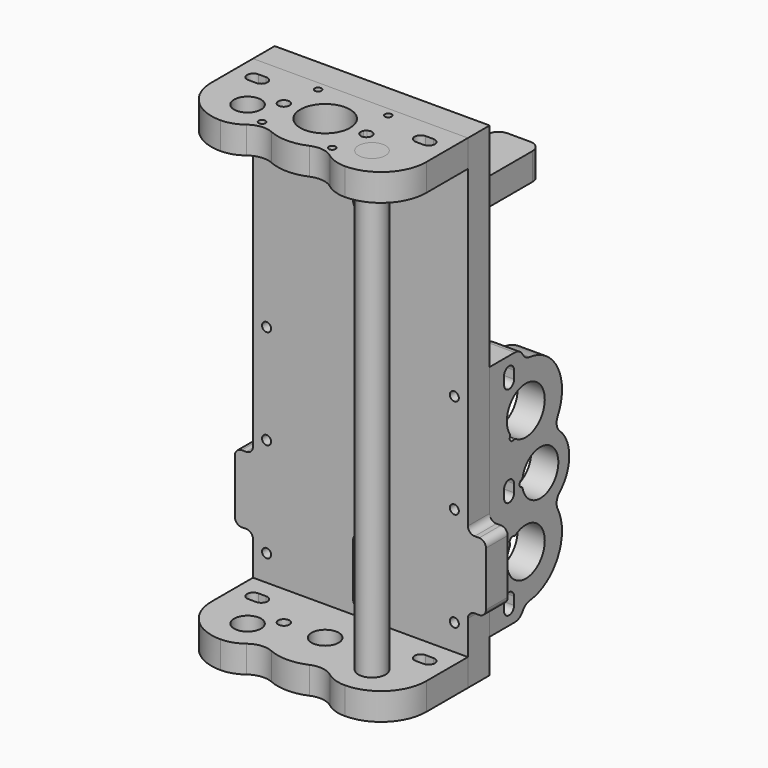
from build123d import *

# Parameters (mm, degrees)
F2_DEPTH       = 12
F3_R           = 11
F3_R_2         = 5.975
F4_DEPTH       = 12
F5_R           = 10
F6_R           = 6
F7_DEPTH       = 214
F9_DEPTH       = 12
F10_R          = 2.5
F10_R_2        = 6
F10_R_3        = 5.9749995874
F11_DEPTH      = 12
F12_R          = 2
F13_DEPTH      = 25
F13_DEPTH_BACK = 10
F14_R          = 1.5
F15_DEPTH      = 25
F16_R          = 5
F17_R          = 5
F18_W          = 8
F18_H          = 30
F19_DEPTH      = 12
F20_R          = 3
F21_W          = 20
F21_H          = 12
F22_DEPTH      = 59
F23_R          = 5


# Not quite as in the source:
# - ends of sketch curves that miss each other by under 0.0002 mm in the source are joined


with BuildPart() as f2:
    # F1 (on Front) → F2 (new body)
    with BuildSketch(Plane.XZ):
        Polygon((-47.5, 1.6334e-06), (47.5, -1.6334e-06), (47.5, 214.0000016334), (-47.5, 214.0000016334), align=None)
        with BuildLine():
            ThreePointArc((3.25, 18), (0, 14.75), (-3.25, 18))
            Line((-3.25, 18), (-3.25, 41))
            ThreePointArc((-3.25, 41), (0, 44.25), (3.25, 41))
            Line((3.25, 41), (3.25, 18))
        make_face(mode=Mode.SUBTRACT)
        with BuildLine():
            ThreePointArc((-3.25, 196.0000016334), (0, 199.2500016334), (3.25, 196.0000016334))
            Line((3.25, 196.0000016334), (3.25, 173.0000016334))
            ThreePointArc((3.25, 173.0000016334), (0, 169.7500016334), (-3.25, 173.0000016334))
            Line((-3.25, 173.0000016334), (-3.25, 196.0000016334))
        make_face(mode=Mode.SUBTRACT)
    extrude(amount=-F2_DEPTH)


with BuildPart() as f4:
    # F3 (on face) → F4 (new body)
    with BuildSketch(Plane.XY.offset(214.0000016334)):
        with BuildLine():
            Line((-7.7942286341, 0), (-47.5, 0))
            Line((-47.5, 0), (-47.5, -23))
            ThreePointArc((-47.5, -23), (-41.6421356237, -37.1421356237), (-27.5, -43))
            ThreePointArc((-27.5, -43), (-42.0543335736, -24.3707612055), (-20.4571797288, -14.7561832304))
            ThreePointArc((-20.4571797288, -14.7561832304), (-15.9364912858, -5.8241729502), (-7.7942286341, 0))
        make_face()
        with BuildLine():
            ThreePointArc((-38.75, -13.5), (-41.5, -10.75), (-38.75, -8))
            Line((-38.75, -8), (-35.25, -8))
            ThreePointArc((-35.25, -8), (-32.5, -10.75), (-35.25, -13.5))
            Line((-35.25, -13.5), (-38.75, -13.5))
        make_face(mode=Mode.SUBTRACT)
        with BuildLine():
            Line((7.7942286341, 0), (-7.7942286341, 0))
            ThreePointArc((-7.7942286341, 0), (-15.9364912858, -5.8241729502), (-20.4571797288, -14.7561832304))
            ThreePointArc((-20.4571797288, -14.7561832304), (-18.5664260205, -15.950466567), (-16.8742462967, -17.4125849124))
            ThreePointArc((-16.8742462967, -17.4125849124), (-16.4091811981, -17.8084367766), (-16.0539715251, -18.3052368697))
            ThreePointArc((-16.0539715251, -18.3052368697), (-13.4164914328, -22.8371726314), (-12.5, -28))
            ThreePointArc((-12.5, -28), (-12.9343908099, -31.5837171931), (-14.212403856, -34.9598698777))
            ThreePointArc((-14.212403856, -34.9598698777), (0, -40.5), (14.212403856, -34.9598698777))
            ThreePointArc((14.212403856, -34.9598698777), (12.5908669986, -26.3514390682), (16.0539715251, -18.3052368697))
            ThreePointArc((16.0539715251, -18.3052368697), (16.4091811981, -17.8084367766), (16.8742462967, -17.4125849124))
            ThreePointArc((16.8742462967, -17.4125849124), (18.5664260205, -15.950466567), (20.4571797288, -14.7561832304))
            ThreePointArc((20.4571797288, -14.7561832304), (15.9364912858, -5.8241729502), (7.7942286341, 0))
        make_face()
        with Locations((0, -19.5)):
            Circle(F3_R, mode=Mode.SUBTRACT)
        with BuildLine():
            Line((47.5, 0), (7.7942286341, 0))
            ThreePointArc((7.7942286341, 0), (15.9364912858, -5.8241729502), (20.4571797288, -14.7561832304))
            ThreePointArc((20.4571797288, -14.7561832304), (35.2252086034, -15.1422726723), (42.5, -28))
            ThreePointArc((42.5, -28), (38.1066017178, -38.6066017178), (27.5, -43))
            ThreePointArc((27.5, -43), (41.6421356237, -37.1421356237), (47.5, -23))
            Line((47.5, -23), (47.5, 0))
        make_face()
        with BuildLine():
            Line((38.75, -13.5), (35.25, -13.5))
            ThreePointArc((35.25, -13.5), (32.5, -10.75), (35.25, -8))
            Line((35.25, -8), (38.75, -8))
            ThreePointArc((38.75, -8), (41.5, -10.75), (38.75, -13.5))
        make_face(mode=Mode.SUBTRACT)
        with BuildLine():
            ThreePointArc((-16.8742462967, -17.4125849124), (-18.5664260205, -15.950466567), (-20.4571797288, -14.7561832304))
            ThreePointArc((-20.4571797288, -14.7561832304), (-20.0634554606, -25.7014316878), (-14.212403856, -34.9598698777))
            ThreePointArc((-14.212403856, -34.9598698777), (-12.9343908099, -31.5837171931), (-12.5, -28))
            ThreePointArc((-12.5, -28), (-13.4164914328, -22.8371726314), (-16.0539715251, -18.3052368697))
            ThreePointArc((-16.0539715251, -18.3052368697), (-15.8271843666, -18.8835874706), (-15.75, -19.5))
            ThreePointArc((-15.75, -19.5), (-20.4510661347, -20.6854568195), (-16.8742462967, -17.4125849124))
        make_face()
        with BuildLine():
            ThreePointArc((-14.212403856, -34.9598698777), (-20.0634554606, -25.7014316878), (-20.4571797288, -14.7561832304))
            ThreePointArc((-20.4571797288, -14.7561832304), (-42.0543335736, -24.3707612055), (-27.5, -43))
            ThreePointArc((-27.5, -43), (-19.7346296986, -40.8335117595), (-14.212403856, -34.9598698777))
        make_face()
        with Locations((-27.5, -28)):
            Circle(F3_R_2, mode=Mode.SUBTRACT)
        with BuildLine():
            ThreePointArc((42.5, -28), (35.2252086034, -15.1422726723), (20.4571797288, -14.7561832304))
            ThreePointArc((20.4571797288, -14.7561832304), (20.0634554606, -25.7014316878), (14.212403856, -34.9598698777))
            ThreePointArc((14.212403856, -34.9598698777), (19.7346296986, -40.8335117595), (27.5, -43))
            ThreePointArc((27.5, -43), (38.1066017178, -38.6066017178), (42.5, -28))
        make_face()
        with Locations((27.5, -28)):
            Circle(F3_R_2, mode=Mode.SUBTRACT)
        with BuildLine():
            ThreePointArc((14.212403856, -34.9598698777), (20.0634554606, -25.7014316878), (20.4571797288, -14.7561832304))
            ThreePointArc((20.4571797288, -14.7561832304), (18.5664260205, -15.950466567), (16.8742462967, -17.4125849124))
            ThreePointArc((16.8742462967, -17.4125849124), (19.4354568195, -17.2989338653), (20.75, -19.5))
            ThreePointArc((20.75, -19.5), (17.6335874706, -21.9228156334), (16.0539715251, -18.3052368697))
            ThreePointArc((16.0539715251, -18.3052368697), (12.5908669986, -26.3514390682), (14.212403856, -34.9598698777))
        make_face()
    extrude(amount=-F4_DEPTH)

    # F5
    f5_edges = [f4.edges().sort_by_distance(p)[0] for p in [
        (-14.212404, -34.95987, 208.000002),
        (14.212404, -34.95987, 208.000002),
    ]]
    fillet(f5_edges, radius=F5_R)


with BuildPart() as f7:
    # F6 (on face) → F7 (new body)
    with BuildSketch(Plane.XY.offset(214.0000016334)):
        with Locations((27.5, -28)):
            Circle(F6_R)
    extrude(amount=-F7_DEPTH)


with BuildPart() as f9:
    # F8 (on face) → F9 (new body)
    with BuildSketch(Plane.YZ.offset(47.5)):
        with BuildLine():
            Line((28.5, 14.9999964573), (32, 19.9999983666))
            ThreePointArc((32, 19.9999983666), (46.1421356237, 25.8578627429), (52, 39.9999983666))
            ThreePointArc((52, 39.9999983666), (50.7273420335, 47.0204442471), (47.071333964, 53.1474274897))
            ThreePointArc((47.071333964, 53.1474274897), (56, 67.4999964573), (47.071333964, 81.8525654249))
            ThreePointArc((47.071333964, 81.8525654249), (50.7273420335, 87.9795486675), (52, 94.9999945479))
            ThreePointArc((52, 94.9999945479), (46.1421356237, 109.1421301717), (32, 114.9999945479))
            Line((32, 114.9999945479), (28.5, 119.9999964573))
            Line((28.5, 119.9999964573), (12, 119.9999964573))
            Line((12, 119.9999964573), (12, 14.9999964573))
            Line((12, 14.9999964573), (28.5, 14.9999964573))
        make_face()
        with BuildLine():
            ThreePointArc((20, 25.2499964573), (22.75, 27.9999964573), (25.5, 25.2499964573))
            Line((25.5, 25.2499964573), (25.5, 21.7499964573))
            ThreePointArc((25.5, 21.7499964573), (22.75, 18.9999964573), (20, 21.7499964573))
            Line((20, 21.7499964573), (20, 25.2499964573))
        make_face(mode=Mode.SUBTRACT)
        with BuildLine():
            ThreePointArc((26.2943182564, 48.7846907824), (39.4069435329, 32.5930548337), (23.2153075842, 45.7056801102))
            ThreePointArc((23.2153075842, 45.7056801102), (23.3755438907, 46.2028582229), (23.2632266648, 46.7130019187))
            ThreePointArc((23.2632266648, 46.7130019187), (23.5323962953, 48.4676020713), (25.286996448, 48.7367717018))
            ThreePointArc((25.286996448, 48.7367717018), (25.7971401438, 48.6244544759), (26.2943182564, 48.7846907824))
        make_face(mode=Mode.SUBTRACT)
        with BuildLine():
            Line((20, 65.5727162957), (20, 69.0727162957))
            ThreePointArc((20, 69.0727162957), (22.75, 71.8227162957), (25.5, 69.0727162957))
            Line((25.5, 69.0727162957), (25.5, 65.5727162957))
            ThreePointArc((25.5, 65.5727162957), (22.75, 62.8227162957), (20, 65.5727162957))
        make_face(mode=Mode.SUBTRACT)
        with BuildLine():
            ThreePointArc((30.2641799544, 69.6712709771), (49.975, 67.4999964573), (30.2641799544, 65.3287219374))
            ThreePointArc((30.2641799544, 65.3287219374), (30.0228916348, 65.7894059146), (29.5828947368, 66.0666287667))
            ThreePointArc((29.5828947368, 66.0666287667), (28.525, 67.4999964573), (29.5828947368, 68.9333641478))
            ThreePointArc((29.5828947368, 68.9333641478), (30.0228916348, 69.210587), (30.2641799544, 69.6712709771))
        make_face(mode=Mode.SUBTRACT)
        with BuildLine():
            Line((25.5, 113.2499964573), (25.5, 109.7499964573))
            ThreePointArc((25.5, 109.7499964573), (22.75, 106.9999964573), (20, 109.7499964573))
            Line((20, 109.7499964573), (20, 113.2499964573))
            ThreePointArc((20, 113.2499964573), (22.75, 115.9999964573), (25.5, 113.2499964573))
        make_face(mode=Mode.SUBTRACT)
        with BuildLine():
            ThreePointArc((23.2632266648, 88.2869909959), (23.3755438907, 88.7971346917), (23.2153075842, 89.2943128043))
            ThreePointArc((23.2153075842, 89.2943128043), (39.4069435329, 102.4069380809), (26.2943182564, 86.2153021321))
            ThreePointArc((26.2943182564, 86.2153021321), (25.7971401438, 86.3755384387), (25.286996448, 86.2632212128))
            ThreePointArc((25.286996448, 86.2632212128), (23.5323962953, 86.5323908432), (23.2632266648, 88.2869909959))
        make_face(mode=Mode.SUBTRACT)
    extrude(amount=-F9_DEPTH)


with BuildPart() as f11:
    # F10 (on face) → F11 (new body)
    with BuildSketch(Plane(origin=(0, 0, 0), x_dir=(1, 0, -3.44e-08), z_dir=(-3.44e-08, 0, -1))):
        with BuildLine():
            Line((-47.5000069462, 23), (-47.5000069462, 0))
            Line((-47.5000069462, 0), (47.4999930538, 0))
            Line((47.4999930538, 0), (47.4999930538, 23))
            ThreePointArc((47.4999930538, 23), (41.6421286776, 37.1421356237), (27.4999930538, 43))
            ThreePointArc((27.4999930538, 43), (22.7171725023, 42.217054249), (18.4336441907, 39.9499508691))
            ThreePointArc((18.4336441907, 39.9499508691), (13.5760949869, 37.9872452657), (8.3928250358, 38.7499445297))
            ThreePointArc((8.3928250358, 38.7499445297), (-7.3588e-06, 40.5), (-8.3928397534, 38.7499445297))
            ThreePointArc((-8.3928397534, 38.7499445297), (-13.5761097045, 37.9872452657), (-18.4336589083, 39.9499508691))
            ThreePointArc((-18.4336589083, 39.9499508691), (-22.7171872199, 42.217054249), (-27.5000073588, 43))
            ThreePointArc((-27.5000073588, 43), (-41.6421425699, 37.1421356237), (-47.5000069462, 23))
        make_face()
        with BuildLine():
            Line((-35.2500069462, 8), (-38.7500069462, 8))
            ThreePointArc((-38.7500069462, 8), (-41.5000069462, 10.75), (-38.7500069462, 13.5))
            Line((-38.7500069462, 13.5), (-35.2500069462, 13.5))
            ThreePointArc((-35.2500069462, 13.5), (-32.5000069462, 10.75), (-35.2500069462, 8))
        make_face(mode=Mode.SUBTRACT)
        with Locations((-18.2500073588, 19.5)):
            Circle(F10_R, mode=Mode.SUBTRACT)
        with Locations((-7.3588e-06, 19.5)):
            Circle(F10_R_2, mode=Mode.SUBTRACT)
        with Locations((18.2499926412, 19.5)):
            Circle(F10_R, mode=Mode.SUBTRACT)
        with BuildLine():
            ThreePointArc((35.2499930538, 8), (32.4999930538, 10.75), (35.2499930538, 13.5))
            Line((35.2499930538, 13.5), (38.7499930538, 13.5))
            ThreePointArc((38.7499930538, 13.5), (41.4999930538, 10.75), (38.7499930538, 8))
            Line((38.7499930538, 8), (35.2499930538, 8))
        make_face(mode=Mode.SUBTRACT)
        with Locations((-27.5000073588, 28)):
            Circle(F10_R_3, mode=Mode.SUBTRACT)
        with Locations((27.4999926412, 28)):
            Circle(F10_R_3, mode=Mode.SUBTRACT)
    extrude(amount=-F11_DEPTH)


with BuildPart() as f13_tool:
    # F12 (on face) → F13 (new body, two sides)
    with BuildSketch(Plane(origin=(0, 12, 0), x_dir=(-1, 0, 0), z_dir=(0, 1, 0))) as f13_sk:
        with Locations((-37, 208.0000016334)):
            Circle(F12_R)
        with Locations((37, 208.0000016334)):
            Circle(F12_R)
        with Locations((37, 6.0000016334)):
            Circle(F12_R)
        with Locations((-37, 6.0000016334)):
            Circle(F12_R)
        with Locations((-41.5, 23.4999987879)):
            Circle(F12_R)
        with Locations((-41.5, 111.4999987879)):
            Circle(F12_R)
        with Locations((-41.5, 67.4999987879)):
            Circle(F12_R)
        with Locations((41.5, 23.4999987879)):
            Circle(F12_R)
        with Locations((41.5, 111.4999987879)):
            Circle(F12_R)
        with Locations((41.5, 67.4999987879)):
            Circle(F12_R)
    extrude(amount=-F13_DEPTH)
    extrude(f13_sk.sketch, amount=F13_DEPTH_BACK)


with BuildPart() as f2_1:
    add(f2.part)

    # F13: cut by f13_tool
    add(f13_tool.part, mode=Mode.SUBTRACT)

    # F18 (on face) → F19 (join)
    with BuildSketch(Plane(origin=(0, 12, 0), x_dir=(-1, 0, 0), z_dir=(0, 1, 0))):
        with Locations((51.5, 45.0000012121)):
            Rectangle(F18_W, F18_H)
        with Locations((-51.5, 45.0000012121)):
            Rectangle(F18_W, F18_H)
    extrude(amount=-F19_DEPTH)

    # F20
    f20_edges = [f2_1.edges().sort_by_distance(p)[0] for p in [
        (-47.5, 6, 60.000001),
        (-47.5, 6, 30.000001),
        (-55.5, 6, 30.000001),
        (-55.5, 6, 60.000001),
        (55.5, 6, 30.000001),
        (47.5, 6, 30.000001),
        (55.5, 6, 60.000001),
        (47.5, 6, 60.000001),
    ]]
    fillet(f20_edges, radius=F20_R)


with BuildPart() as f4_1:
    add(f4.part)

    # F13: cut by f13_tool
    add(f13_tool.part, mode=Mode.SUBTRACT)

    # F14 (on face) → F15 (cut)
    with BuildSketch(Plane.XY.offset(214.0000016334)):
        with Locations((-15.5, -4)):
            Circle(F14_R)
        with Locations((-15.5, -35)):
            Circle(F14_R)
        with Locations((15.5, -35)):
            Circle(F14_R)
        with Locations((15.5, -4)):
            Circle(F14_R)
    extrude(amount=-F15_DEPTH, mode=Mode.SUBTRACT)


with BuildPart() as f9_1:
    add(f9.part)

    # F13: cut by f13_tool
    add(f13_tool.part, mode=Mode.SUBTRACT)

    # F16
    f16_edges = [f9_1.edges().sort_by_distance(p)[0] for p in [
        (41.5, 32, 19.999998),
        (41.5, 28.5, 14.999996),
        (41.5, 32, 114.999995),
        (41.5, 28.5, 119.999996),
    ]]
    fillet(f16_edges, radius=F16_R)

    # F17
    f17_edges = [f9_1.edges().sort_by_distance(p)[0] for p in [
        (41.5, 47.071334, 81.852565),
        (41.5, 47.071334, 53.147427),
    ]]
    fillet(f17_edges, radius=F17_R)


with BuildPart() as f11_1:
    add(f11.part)

    # F13: cut by f13_tool
    add(f13_tool.part, mode=Mode.SUBTRACT)


with BuildPart() as f22:
    # F21 (on face) → F22 (new body)
    with BuildSketch(Plane(origin=(0, 12, 0), x_dir=(-1, 0, 0), z_dir=(0, 1, 0))):
        with Locations((-13.25, 168.1933916334)):
            Rectangle(F21_W, F21_H)
    extrude(amount=F22_DEPTH)

    # F23
    f23_edges = [f22.edges().sort_by_distance(p)[0] for p in [
        (3.25, 71, 168.193392),
        (23.25, 71, 168.193392),
    ]]
    fillet(f23_edges, radius=F23_R)


solid = Compound([f7.part, f2_1.part, f4_1.part, f9_1.part, f11_1.part, f22.part])
